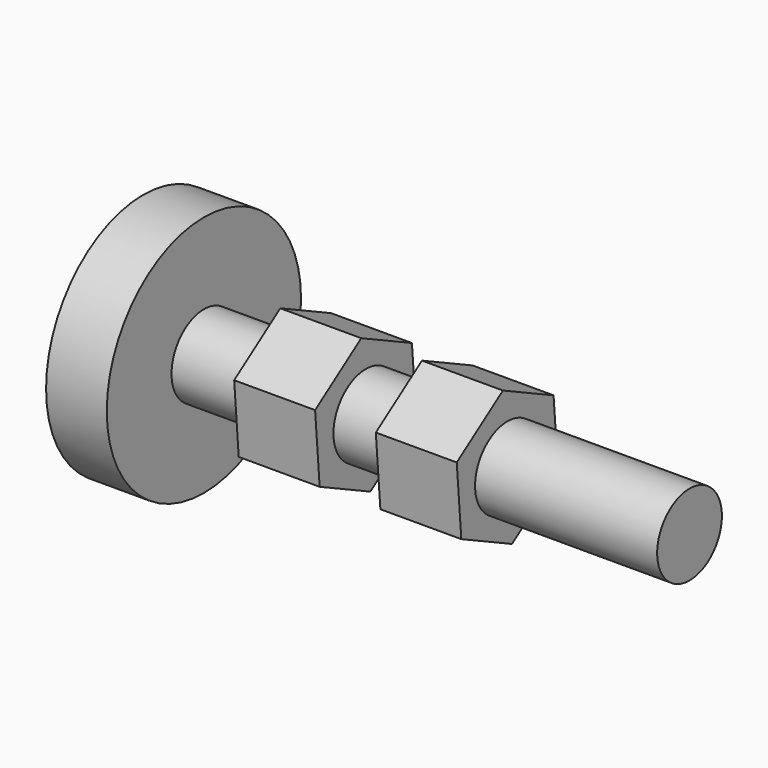
from build123d import *

# Parameters (mm, degrees)
F0_R     = 19.05
F1_DEPTH = 9.525
F2_R     = 6.35
F3_DEPTH = 76.2
F5_DEPTH = 12.7
F6_R     = 6.35
F7_DEPTH = 22.226


with BuildPart() as f1:
    # F0 (on Right) → F1 (new body)
    with BuildSketch(Plane.YZ):
        Circle(F0_R)
    extrude(amount=-F1_DEPTH)

    # F2 (on face) → F3 (join)
    with BuildSketch(Plane.YZ):
        Circle(F2_R)
    extrude(amount=F3_DEPTH)


with BuildPart() as f5:
    # F4 (on Right) → F5 (new body)
    with BuildSketch(Plane.YZ):
        Polygon((-0.8951443086, 10.9620352429), (-9.9409731518, 4.7057999102), (-9.0458288433, -6.2562353327), (0.8951443086, -10.9620352429), (9.9409731518, -4.7057999102), (9.0458288433, 6.2562353327), align=None)
    extrude(amount=F5_DEPTH)

    # F6 (on face) → F7 (cut, through all)
    with BuildSketch(Plane.YZ.offset(12.7)):
        Circle(F6_R)
    extrude(amount=-F7_DEPTH, mode=Mode.SUBTRACT)


with BuildPart() as f5_1:
    # F8: moved
    add(f5.part.moved(Location((12.7, 0, 0))))


with BuildPart() as f9_1:
    # F9: copy of F5
    add(f5_1.part.moved(Location((22.225, 0, 0))))


solid = Compound([f1.part, f5_1.part, f9_1.part])
